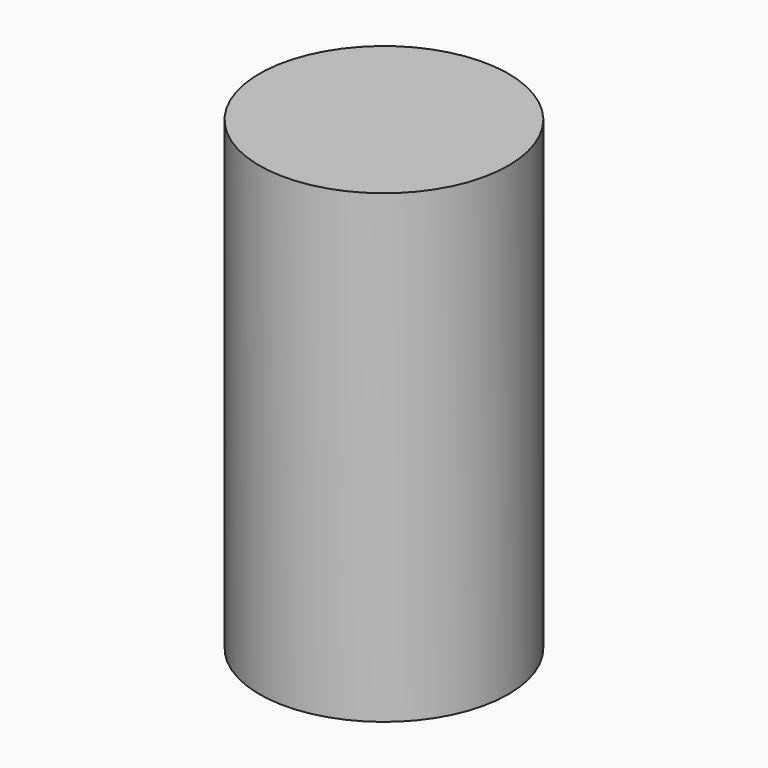
from build123d import *

# Parameters (mm, degrees)
F0_R     = 40.765916218
F1_DEPTH = 152.4


# Not quite as in the source:
# - a feature names something its author has since deleted; it is built from what else it names


with BuildPart() as f1:
    # F0 (on Top) → F1 (new body)
    with BuildSketch(Plane.XY):
        Circle(F0_R)
    extrude(amount=F1_DEPTH)


solid = f1.part
